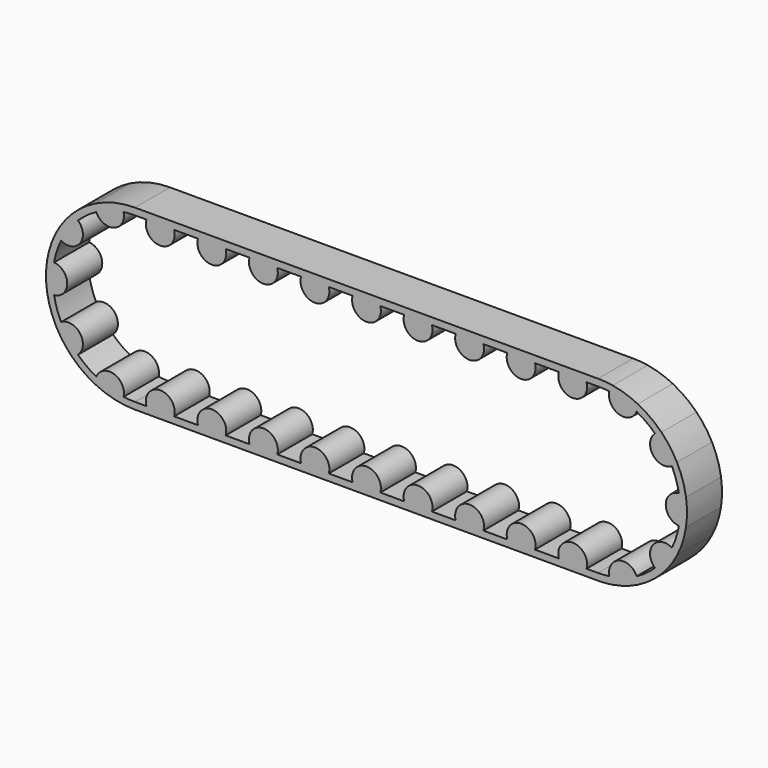
from build123d import *

# Parameters (mm, degrees)
F3_DEPTH = 25.4


with BuildPart() as f3:
    # F2 (on Front) → F3 (new body)
    with BuildSketch(Plane.XZ):
        with BuildLine():
            ThreePointArc((-6.5580901404, 47.171305671), (-3.2868824452, 47.5114410305), (0, 47.625))
            Line((0, 47.625), (6.6759446819, 47.625))
            ThreePointArc((6.6759446819, 47.625), (7.6523000339, 49.786472114), (9.1956373991, 51.5874))
            Line((9.1956373991, 51.5874), (0, 51.5874))
            ThreePointArc((0, 51.5874), (-4.2571154541, 51.4114462622), (-8.485190663, 50.8847853309))
            ThreePointArc((-8.485190663, 50.8847853309), (-7.2859359113, 49.1503637276), (-6.5580901404, 47.171305671))
        make_face()
        with BuildLine():
            ThreePointArc((9.1956373991, 51.5874), (7.6523000339, 49.786472114), (6.6759446819, 47.625))
            Line((6.6759446819, 47.625), (22.7579240323, 47.625))
            ThreePointArc((22.7579240323, 47.625), (21.7815686803, 49.786472114), (20.2382313151, 51.5874))
            Line((20.2382313151, 51.5874), (9.1956373991, 51.5874))
        make_face()
        with BuildLine():
            Line((22.7579240323, 47.625), (6.6759446819, 47.625))
            ThreePointArc((6.6759446819, 47.625), (14.7169343571, 36.9220438028), (22.7579240323, 47.625))
        make_face()
        with BuildLine():
            ThreePointArc((-22.4209914306, 42.0171366024), (-12.129837039, 37.3317997636), (-6.5580901404, 47.171305671))
            ThreePointArc((-6.5580901404, 47.171305671), (-14.7169343571, 45.2940665886), (-22.4209914306, 42.0171366024))
        make_face()
        with BuildLine():
            ThreePointArc((-22.4209914306, 42.0171366024), (-14.7169343571, 45.2940665886), (-6.5580901404, 47.171305671))
            ThreePointArc((-6.5580901404, 47.171305671), (-7.2859359113, 49.1503637276), (-8.485190663, 50.8847853309))
            ThreePointArc((-8.485190663, 50.8847853309), (-15.9413832956, 49.0625329287), (-23.0446629367, 46.1541260224))
            ThreePointArc((-23.0446629367, 46.1541260224), (-22.9954129717, 44.0460452131), (-22.4209914306, 42.0171366024))
        make_face()
        with BuildLine():
            ThreePointArc((20.2382313151, 51.5874), (21.7815686803, 49.786472114), (22.7579240323, 47.625))
            Line((22.7579240323, 47.625), (36.5771902535, 47.625))
            ThreePointArc((36.5771902535, 47.625), (37.5535456055, 49.786472114), (39.0968829707, 51.5874))
            Line((39.0968829707, 51.5874), (20.2382313151, 51.5874))
        make_face()
        with BuildLine():
            ThreePointArc((-33.032204179, 34.307639267), (-27.9932726404, 38.5294343571), (-22.4209914306, 42.0171366024))
            ThreePointArc((-22.4209914306, 42.0171366024), (-22.9954129717, 44.0460452131), (-23.0446629367, 46.1541260224))
            ThreePointArc((-23.0446629367, 46.1541260224), (-30.3223129241, 41.7350832956), (-36.7739898304, 36.1791861533))
            ThreePointArc((-36.7739898304, 36.1791861533), (-34.7843049161, 35.4809138575), (-33.032204179, 34.307639267))
        make_face()
        with BuildLine():
            ThreePointArc((39.0968829707, 51.5874), (37.5535456055, 49.786472114), (36.5771902535, 47.625))
            Line((36.5771902535, 47.625), (52.6591696039, 47.625))
            ThreePointArc((52.6591696039, 47.625), (51.6828142519, 49.786472114), (50.1394768867, 51.5874))
            Line((50.1394768867, 51.5874), (39.0968829707, 51.5874))
        make_face()
        with BuildLine():
            Line((52.6591696039, 47.625), (36.5771902535, 47.625))
            ThreePointArc((36.5771902535, 47.625), (44.6181799287, 36.9220438028), (52.6591696039, 47.625))
        make_face()
        with BuildLine():
            ThreePointArc((-42.8360163366, 20.8138494617), (-31.7563256461, 23.0723211151), (-33.032204179, 34.307639267))
            ThreePointArc((-33.032204179, 34.307639267), (-38.5294343571, 27.9932726404), (-42.8360163366, 20.8138494617))
        make_face()
        with BuildLine():
            ThreePointArc((-42.8360163366, 20.8138494617), (-38.5294343571, 27.9932726404), (-33.032204179, 34.307639267))
            ThreePointArc((-33.032204179, 34.307639267), (-34.7843049161, 35.4809138575), (-36.7739898304, 36.1791861533))
            ThreePointArc((-36.7739898304, 36.1791861533), (-41.7350832956, 30.3223129241), (-45.7722385539, 23.7941592944))
            ThreePointArc((-45.7722385539, 23.7941592944), (-44.4932956849, 22.1176344973), (-42.8360163366, 20.8138494617))
        make_face()
        with BuildLine():
            ThreePointArc((50.1394768867, 51.5874), (51.6828142519, 49.786472114), (52.6591696039, 47.625))
            Line((52.6591696039, 47.625), (66.478435825, 47.625))
            ThreePointArc((66.478435825, 47.625), (67.4547911771, 49.786472114), (68.9981285423, 51.5874))
            Line((68.9981285423, 51.5874), (50.1394768867, 51.5874))
        make_face()
        with BuildLine():
            ThreePointArc((-46.8891389446, 8.3396207368), (-45.2940665886, 14.7169343571), (-42.8360163366, 20.8138494617))
            ThreePointArc((-42.8360163366, 20.8138494617), (-44.4932956849, 22.1176344973), (-45.7722385539, 23.7941592944))
            ThreePointArc((-45.7722385539, 23.7941592944), (-49.0625329287, 15.9413832956), (-51.0163747846, 7.6543675504))
            ThreePointArc((-51.0163747846, 7.6543675504), (-48.9962517179, 8.2589608458), (-46.8891389446, 8.3396207368))
        make_face()
        with BuildLine():
            ThreePointArc((68.9981285423, 51.5874), (67.4547911771, 49.786472114), (66.478435825, 47.625))
            Line((66.478435825, 47.625), (82.5604151755, 47.625))
            ThreePointArc((82.5604151755, 47.625), (81.5840598235, 49.786472114), (80.0407224583, 51.5874))
            Line((80.0407224583, 51.5874), (68.9981285423, 51.5874))
        make_face()
        with BuildLine():
            Line((82.5604151755, 47.625), (66.478435825, 47.625))
            ThreePointArc((66.478435825, 47.625), (74.5194255003, 36.9220438028), (82.5604151755, 47.625))
        make_face()
        with BuildLine():
            ThreePointArc((-46.8891389446, -8.3396207368), (-39.2529772142, 0), (-46.8891389446, 8.3396207368))
            ThreePointArc((-46.8891389446, 8.3396207368), (-47.625, 0), (-46.8891389446, -8.3396207368))
        make_face()
        with BuildLine():
            ThreePointArc((-46.8891389446, -8.3396207368), (-47.625, 0), (-46.8891389446, 8.3396207368))
            ThreePointArc((-46.8891389446, 8.3396207368), (-48.9962517179, 8.2589608458), (-51.0163747846, 7.6543675504))
            ThreePointArc((-51.0163747846, 7.6543675504), (-51.5874, 0), (-51.0163747846, -7.6543675504))
            ThreePointArc((-51.0163747846, -7.6543675504), (-48.9962517179, -8.2589608458), (-46.8891389446, -8.3396207368))
        make_face()
        with BuildLine():
            ThreePointArc((80.0407224583, 51.5874), (81.5840598235, 49.786472114), (82.5604151755, 47.625))
            Line((82.5604151755, 47.625), (96.3796813966, 47.625))
            ThreePointArc((96.3796813966, 47.625), (97.3560367487, 49.786472114), (98.8993741139, 51.5874))
            Line((98.8993741139, 51.5874), (80.0407224583, 51.5874))
        make_face()
        with BuildLine():
            ThreePointArc((-42.8360163366, -20.8138494617), (-45.2940665886, -14.7169343571), (-46.8891389446, -8.3396207368))
            ThreePointArc((-46.8891389446, -8.3396207368), (-48.9962517179, -8.2589608458), (-51.0163747846, -7.6543675504))
            ThreePointArc((-51.0163747846, -7.6543675504), (-49.0625329287, -15.9413832956), (-45.7722385539, -23.7941592944))
            ThreePointArc((-45.7722385539, -23.7941592944), (-44.4932956849, -22.1176344973), (-42.8360163366, -20.8138494617))
        make_face()
        with BuildLine():
            ThreePointArc((98.8993741139, 51.5874), (97.3560367487, 49.786472114), (96.3796813966, 47.625))
            Line((96.3796813966, 47.625), (112.4616607471, 47.625))
            ThreePointArc((112.4616607471, 47.625), (111.485305395, 49.786472114), (109.9419680298, 51.5874))
            Line((109.9419680298, 51.5874), (98.8993741139, 51.5874))
        make_face()
        with BuildLine():
            Line((112.4616607471, 47.625), (96.3796813966, 47.625))
            ThreePointArc((96.3796813966, 47.625), (104.4206710719, 36.9220438028), (112.4616607471, 47.625))
        make_face()
        with BuildLine():
            ThreePointArc((-33.032204179, -34.307639267), (-31.7563256461, -23.0723211151), (-42.8360163366, -20.8138494617))
            ThreePointArc((-42.8360163366, -20.8138494617), (-38.5294343571, -27.9932726404), (-33.032204179, -34.307639267))
        make_face()
        with BuildLine():
            ThreePointArc((-33.032204179, -34.307639267), (-38.5294343571, -27.9932726404), (-42.8360163366, -20.8138494617))
            ThreePointArc((-42.8360163366, -20.8138494617), (-44.4932956849, -22.1176344973), (-45.7722385539, -23.7941592944))
            ThreePointArc((-45.7722385539, -23.7941592944), (-41.7350832956, -30.3223129241), (-36.7739898304, -36.1791861533))
            ThreePointArc((-36.7739898304, -36.1791861533), (-34.7843049161, -35.4809138575), (-33.032204179, -34.307639267))
        make_face()
        with BuildLine():
            ThreePointArc((109.9419680298, 51.5874), (111.485305395, 49.786472114), (112.4616607471, 47.625))
            Line((112.4616607471, 47.625), (126.2809269682, 47.625))
            ThreePointArc((126.2809269682, 47.625), (127.2572823202, 49.786472114), (128.8006196855, 51.5874))
            Line((128.8006196855, 51.5874), (109.9419680298, 51.5874))
        make_face()
        with BuildLine():
            ThreePointArc((-22.4209914306, -42.0171366024), (-27.9932726404, -38.5294343571), (-33.032204179, -34.307639267))
            ThreePointArc((-33.032204179, -34.307639267), (-34.7843049161, -35.4809138575), (-36.7739898304, -36.1791861533))
            ThreePointArc((-36.7739898304, -36.1791861533), (-30.3223129241, -41.7350832956), (-23.0446629367, -46.1541260224))
            ThreePointArc((-23.0446629367, -46.1541260224), (-22.9954129717, -44.0460452131), (-22.4209914306, -42.0171366024))
        make_face()
        with BuildLine():
            ThreePointArc((128.8006196855, 51.5874), (127.2572823202, 49.786472114), (126.2809269682, 47.625))
            Line((126.2809269682, 47.625), (142.3629063187, 47.625))
            ThreePointArc((142.3629063187, 47.625), (141.3865509666, 49.786472114), (139.8432136014, 51.5874))
            Line((139.8432136014, 51.5874), (128.8006196855, 51.5874))
        make_face()
        with BuildLine():
            Line((142.3629063187, 47.625), (126.2809269682, 47.625))
            ThreePointArc((126.2809269682, 47.625), (134.3219166434, 36.9220438028), (142.3629063187, 47.625))
        make_face()
        with BuildLine():
            ThreePointArc((-6.5580901404, -47.171305671), (-12.129837039, -37.3317997636), (-22.4209914306, -42.0171366024))
            ThreePointArc((-22.4209914306, -42.0171366024), (-14.7169343571, -45.2940665886), (-6.5580901404, -47.171305671))
        make_face()
        with BuildLine():
            ThreePointArc((-6.5580901404, -47.171305671), (-14.7169343571, -45.2940665886), (-22.4209914306, -42.0171366024))
            ThreePointArc((-22.4209914306, -42.0171366024), (-22.9954129717, -44.0460452131), (-23.0446629367, -46.1541260224))
            ThreePointArc((-23.0446629367, -46.1541260224), (-15.9413832956, -49.0625329287), (-8.485190663, -50.8847853309))
            ThreePointArc((-8.485190663, -50.8847853309), (-7.2859359113, -49.1503637276), (-6.5580901404, -47.171305671))
        make_face()
        with BuildLine():
            ThreePointArc((139.8432136014, 51.5874), (141.3865509666, 49.786472114), (142.3629063187, 47.625))
            Line((142.3629063187, 47.625), (156.1821725398, 47.625))
            ThreePointArc((156.1821725398, 47.625), (157.1585278918, 49.786472114), (158.701865257, 51.5874))
            Line((158.701865257, 51.5874), (139.8432136014, 51.5874))
        make_face()
        with BuildLine():
            ThreePointArc((0, -47.625), (-3.2868824452, -47.5114410305), (-6.5580901404, -47.171305671))
            ThreePointArc((-6.5580901404, -47.171305671), (-7.2859359113, -49.1503637276), (-8.485190663, -50.8847853309))
            ThreePointArc((-8.485190663, -50.8847853309), (-4.2571154541, -51.4114462622), (0, -51.5874))
            Line((0, -51.5874), (9.1956373991, -51.5874))
            ThreePointArc((9.1956373991, -51.5874), (7.6523000339, -49.786472114), (6.6759446819, -47.625))
            Line((6.6759446819, -47.625), (0, -47.625))
        make_face()
        with BuildLine():
            ThreePointArc((158.701865257, 51.5874), (157.1585278918, 49.786472114), (156.1821725398, 47.625))
            Line((156.1821725398, 47.625), (172.2641518903, 47.625))
            ThreePointArc((172.2641518903, 47.625), (171.2877965382, 49.786472114), (169.744459173, 51.5874))
            Line((169.744459173, 51.5874), (158.701865257, 51.5874))
        make_face()
        with BuildLine():
            Line((172.2641518903, 47.625), (156.1821725398, 47.625))
            ThreePointArc((156.1821725398, 47.625), (164.223162215, 36.9220438028), (172.2641518903, 47.625))
        make_face()
        with BuildLine():
            ThreePointArc((169.744459173, 51.5874), (171.2877965382, 49.786472114), (172.2641518903, 47.625))
            Line((172.2641518903, 47.625), (186.0834181114, 47.625))
            ThreePointArc((186.0834181114, 47.625), (187.0597734634, 49.786472114), (188.6031108286, 51.5874))
            Line((188.6031108286, 51.5874), (169.744459173, 51.5874))
        make_face()
        with BuildLine():
            ThreePointArc((22.7579240323, -47.625), (14.7169343571, -36.9220438028), (6.6759446819, -47.625))
            Line((6.6759446819, -47.625), (22.7579240323, -47.625))
        make_face()
        with BuildLine():
            Line((22.7579240323, -47.625), (6.6759446819, -47.625))
            ThreePointArc((6.6759446819, -47.625), (7.6523000339, -49.786472114), (9.1956373991, -51.5874))
            Line((9.1956373991, -51.5874), (20.2382313151, -51.5874))
            ThreePointArc((20.2382313151, -51.5874), (21.7815686803, -49.786472114), (22.7579240323, -47.625))
        make_face()
        with BuildLine():
            ThreePointArc((188.6031108286, 51.5874), (187.0597734634, 49.786472114), (186.0834181114, 47.625))
            Line((186.0834181114, 47.625), (202.1653974618, 47.625))
            Line((202.1653974618, 47.625), (215.984663683, 47.625))
            ThreePointArc((215.984663683, 47.625), (216.961019035, 49.786472114), (218.5043564002, 51.5874))
            Line((218.5043564002, 51.5874), (188.6031108286, 51.5874))
        make_face()
        with BuildLine():
            Line((202.1653974618, 47.625), (186.0834181114, 47.625))
            ThreePointArc((186.0834181114, 47.625), (194.1244077866, 36.9220438028), (202.1653974618, 47.625))
        make_face()
        with BuildLine():
            Line((36.5771902535, -47.625), (22.7579240323, -47.625))
            ThreePointArc((22.7579240323, -47.625), (21.7815686803, -49.786472114), (20.2382313151, -51.5874))
            Line((20.2382313151, -51.5874), (39.0968829707, -51.5874))
            ThreePointArc((39.0968829707, -51.5874), (37.5535456055, -49.786472114), (36.5771902535, -47.625))
        make_face()
        with BuildLine():
            ThreePointArc((52.6591696039, -47.625), (44.6181799287, -36.9220438028), (36.5771902535, -47.625))
            Line((36.5771902535, -47.625), (52.6591696039, -47.625))
        make_face()
        with BuildLine():
            Line((52.6591696039, -47.625), (36.5771902535, -47.625))
            ThreePointArc((36.5771902535, -47.625), (37.5535456055, -49.786472114), (39.0968829707, -51.5874))
            Line((39.0968829707, -51.5874), (50.1394768867, -51.5874))
            ThreePointArc((50.1394768867, -51.5874), (51.6828142519, -49.786472114), (52.6591696039, -47.625))
        make_face()
        with BuildLine():
            ThreePointArc((218.5043564002, 51.5874), (216.961019035, 49.786472114), (215.984663683, 47.625))
            Line((215.984663683, 47.625), (232.0666430334, 47.625))
            ThreePointArc((232.0666430334, 47.625), (231.0902876814, 49.786472114), (229.5469503162, 51.5874))
            Line((229.5469503162, 51.5874), (218.5043564002, 51.5874))
        make_face()
        with BuildLine():
            Line((232.0666430334, 47.625), (215.984663683, 47.625))
            ThreePointArc((215.984663683, 47.625), (224.0256533582, 36.9220438028), (232.0666430334, 47.625))
        make_face()
        with BuildLine():
            Line((66.478435825, -47.625), (52.6591696039, -47.625))
            ThreePointArc((52.6591696039, -47.625), (51.6828142519, -49.786472114), (50.1394768867, -51.5874))
            Line((50.1394768867, -51.5874), (68.9981285423, -51.5874))
            ThreePointArc((68.9981285423, -51.5874), (67.4547911771, -49.786472114), (66.478435825, -47.625))
        make_face()
        with BuildLine():
            ThreePointArc((229.5469503162, 51.5874), (231.0902876814, 49.786472114), (232.0666430334, 47.625))
            Line((232.0666430334, 47.625), (245.8859092545, 47.625))
            ThreePointArc((245.8859092545, 47.625), (246.8622646066, 49.786472114), (248.4056019718, 51.5874))
            Line((248.4056019718, 51.5874), (229.5469503162, 51.5874))
        make_face()
        with BuildLine():
            ThreePointArc((82.5604151755, -47.625), (74.5194255003, -36.9220438028), (66.478435825, -47.625))
            Line((66.478435825, -47.625), (82.5604151755, -47.625))
        make_face()
        with BuildLine():
            Line((82.5604151755, -47.625), (66.478435825, -47.625))
            ThreePointArc((66.478435825, -47.625), (67.4547911771, -49.786472114), (68.9981285423, -51.5874))
            Line((68.9981285423, -51.5874), (80.0407224583, -51.5874))
            ThreePointArc((80.0407224583, -51.5874), (81.5840598235, -49.786472114), (82.5604151755, -47.625))
        make_face()
        with BuildLine():
            ThreePointArc((248.4056019718, 51.5874), (246.8622646066, 49.786472114), (245.8859092545, 47.625))
            Line((245.8859092545, 47.625), (261.967888605, 47.625))
            ThreePointArc((261.967888605, 47.625), (260.991533253, 49.786472114), (259.4481958878, 51.5874))
            Line((259.4481958878, 51.5874), (248.4056019718, 51.5874))
        make_face()
        with BuildLine():
            Line((261.967888605, 47.625), (245.8859092545, 47.625))
            ThreePointArc((245.8859092545, 47.625), (253.9268989298, 36.9220438028), (261.967888605, 47.625))
        make_face()
        with BuildLine():
            Line((96.3796813966, -47.625), (82.5604151755, -47.625))
            ThreePointArc((82.5604151755, -47.625), (81.5840598235, -49.786472114), (80.0407224583, -51.5874))
            Line((80.0407224583, -51.5874), (98.8993741139, -51.5874))
            ThreePointArc((98.8993741139, -51.5874), (97.3560367487, -49.786472114), (96.3796813966, -47.625))
        make_face()
        with BuildLine():
            ThreePointArc((259.4481958878, 51.5874), (260.991533253, 49.786472114), (261.967888605, 47.625))
            Line((261.967888605, 47.625), (268.6438332869, 47.625))
            ThreePointArc((268.6438332869, 47.625), (271.930715732, 47.5114410305), (275.2019234272, 47.171305671))
            ThreePointArc((275.2019234272, 47.171305671), (275.9297691982, 49.1503637276), (277.1290239498, 50.8847853309))
            ThreePointArc((277.1290239498, 50.8847853309), (272.900948741, 51.4114462622), (268.6438332869, 51.5874))
            Line((268.6438332869, 51.5874), (259.4481958878, 51.5874))
        make_face()
        with BuildLine():
            ThreePointArc((112.4616607471, -47.625), (104.4206710719, -36.9220438028), (96.3796813966, -47.625))
            Line((96.3796813966, -47.625), (112.4616607471, -47.625))
        make_face()
        with BuildLine():
            Line((112.4616607471, -47.625), (96.3796813966, -47.625))
            ThreePointArc((96.3796813966, -47.625), (97.3560367487, -49.786472114), (98.8993741139, -51.5874))
            Line((98.8993741139, -51.5874), (109.9419680298, -51.5874))
            ThreePointArc((109.9419680298, -51.5874), (111.485305395, -49.786472114), (112.4616607471, -47.625))
        make_face()
        with BuildLine():
            Line((126.2809269682, -47.625), (112.4616607471, -47.625))
            ThreePointArc((112.4616607471, -47.625), (111.485305395, -49.786472114), (109.9419680298, -51.5874))
            Line((109.9419680298, -51.5874), (128.8006196855, -51.5874))
            ThreePointArc((128.8006196855, -51.5874), (127.2572823202, -49.786472114), (126.2809269682, -47.625))
        make_face()
        with BuildLine():
            ThreePointArc((277.1290239498, 50.8847853309), (275.9297691982, 49.1503637276), (275.2019234272, 47.171305671))
            ThreePointArc((275.2019234272, 47.171305671), (283.360767644, 45.2940665886), (291.0648247175, 42.0171366024))
            ThreePointArc((291.0648247175, 42.0171366024), (291.6392462586, 44.0460452131), (291.6884962236, 46.1541260224))
            ThreePointArc((291.6884962236, 46.1541260224), (284.5852165825, 49.0625329287), (277.1290239498, 50.8847853309))
        make_face()
        with BuildLine():
            ThreePointArc((291.0648247175, 42.0171366024), (283.360767644, 45.2940665886), (275.2019234272, 47.171305671))
            ThreePointArc((275.2019234272, 47.171305671), (280.7736703259, 37.3317997636), (291.0648247175, 42.0171366024))
        make_face()
        with BuildLine():
            ThreePointArc((142.3629063187, -47.625), (134.3219166434, -36.9220438028), (126.2809269682, -47.625))
            Line((126.2809269682, -47.625), (142.3629063187, -47.625))
        make_face()
        with BuildLine():
            Line((142.3629063187, -47.625), (126.2809269682, -47.625))
            ThreePointArc((126.2809269682, -47.625), (127.2572823202, -49.786472114), (128.8006196855, -51.5874))
            Line((128.8006196855, -51.5874), (139.8432136014, -51.5874))
            ThreePointArc((139.8432136014, -51.5874), (141.3865509666, -49.786472114), (142.3629063187, -47.625))
        make_face()
        with BuildLine():
            ThreePointArc((291.6884962236, 46.1541260224), (291.6392462586, 44.0460452131), (291.0648247175, 42.0171366024))
            ThreePointArc((291.0648247175, 42.0171366024), (296.6371059273, 38.5294343571), (301.6760374659, 34.307639267))
            ThreePointArc((301.6760374659, 34.307639267), (303.4281382029, 35.4809138575), (305.4178231173, 36.1791861533))
            ThreePointArc((305.4178231173, 36.1791861533), (298.966146211, 41.7350832956), (291.6884962236, 46.1541260224))
        make_face()
        with BuildLine():
            Line((156.1821725398, -47.625), (142.3629063187, -47.625))
            ThreePointArc((142.3629063187, -47.625), (141.3865509666, -49.786472114), (139.8432136014, -51.5874))
            Line((139.8432136014, -51.5874), (158.701865257, -51.5874))
            ThreePointArc((158.701865257, -51.5874), (157.1585278918, -49.786472114), (156.1821725398, -47.625))
        make_face()
        with BuildLine():
            ThreePointArc((305.4178231173, 36.1791861533), (303.4281382029, 35.4809138575), (301.6760374659, 34.307639267))
            ThreePointArc((301.6760374659, 34.307639267), (307.173267644, 27.9932726404), (311.4798496235, 20.8138494617))
            ThreePointArc((311.4798496235, 20.8138494617), (313.1371289717, 22.1176344973), (314.4160718408, 23.7941592944))
            ThreePointArc((314.4160718408, 23.7941592944), (310.3789165825, 30.3223129241), (305.4178231173, 36.1791861533))
        make_face()
        with BuildLine():
            ThreePointArc((311.4798496235, 20.8138494617), (307.173267644, 27.9932726404), (301.6760374659, 34.307639267))
            ThreePointArc((301.6760374659, 34.307639267), (300.400158933, 23.0723211151), (311.4798496235, 20.8138494617))
        make_face()
        with BuildLine():
            ThreePointArc((172.2641518903, -47.625), (164.223162215, -36.9220438028), (156.1821725398, -47.625))
            Line((156.1821725398, -47.625), (172.2641518903, -47.625))
        make_face()
        with BuildLine():
            Line((172.2641518903, -47.625), (156.1821725398, -47.625))
            ThreePointArc((156.1821725398, -47.625), (157.1585278918, -49.786472114), (158.701865257, -51.5874))
            Line((158.701865257, -51.5874), (169.744459173, -51.5874))
            ThreePointArc((169.744459173, -51.5874), (171.2877965382, -49.786472114), (172.2641518903, -47.625))
        make_face()
        with BuildLine():
            ThreePointArc((314.4160718408, 23.7941592944), (313.1371289717, 22.1176344973), (311.4798496235, 20.8138494617))
            ThreePointArc((311.4798496235, 20.8138494617), (313.9378998754, 14.7169343571), (315.5329722315, 8.3396207368))
            ThreePointArc((315.5329722315, 8.3396207368), (317.6400850048, 8.2589608458), (319.6602080715, 7.6543675504))
            ThreePointArc((319.6602080715, 7.6543675504), (317.7063662156, 15.9413832956), (314.4160718408, 23.7941592944))
        make_face()
        with BuildLine():
            Line((186.0834181114, -47.625), (172.2641518903, -47.625))
            ThreePointArc((172.2641518903, -47.625), (171.2877965382, -49.786472114), (169.744459173, -51.5874))
            Line((169.744459173, -51.5874), (188.6031108286, -51.5874))
            ThreePointArc((188.6031108286, -51.5874), (187.0597734634, -49.786472114), (186.0834181114, -47.625))
        make_face()
        with BuildLine():
            ThreePointArc((319.6602080715, 7.6543675504), (317.6400850048, 8.2589608458), (315.5329722315, 8.3396207368))
            ThreePointArc((315.5329722315, 8.3396207368), (316.2688332869, 0), (315.5329722315, -8.3396207368))
            ThreePointArc((315.5329722315, -8.3396207368), (317.6400850048, -8.2589608458), (319.6602080715, -7.6543675504))
            ThreePointArc((319.6602080715, -7.6543675504), (320.2312332869, 0), (319.6602080715, 7.6543675504))
        make_face()
        with BuildLine():
            ThreePointArc((315.5329722315, -8.3396207368), (316.2688332869, 0), (315.5329722315, 8.3396207368))
            ThreePointArc((315.5329722315, 8.3396207368), (307.8968105011, 0), (315.5329722315, -8.3396207368))
        make_face()
        with BuildLine():
            ThreePointArc((202.1653974618, -47.625), (194.1244077866, -36.9220438028), (186.0834181114, -47.625))
            Line((186.0834181114, -47.625), (202.1653974618, -47.625))
        make_face()
        with BuildLine():
            Line((202.1653974618, -47.625), (186.0834181114, -47.625))
            ThreePointArc((186.0834181114, -47.625), (187.0597734634, -49.786472114), (188.6031108286, -51.5874))
            Line((188.6031108286, -51.5874), (199.6457047446, -51.5874))
            ThreePointArc((199.6457047446, -51.5874), (201.1890421098, -49.786472114), (202.1653974618, -47.625))
        make_face()
        with BuildLine():
            ThreePointArc((319.6602080715, -7.6543675504), (317.6400850048, -8.2589608458), (315.5329722315, -8.3396207368))
            ThreePointArc((315.5329722315, -8.3396207368), (313.9378998754, -14.7169343571), (311.4798496235, -20.8138494617))
            ThreePointArc((311.4798496235, -20.8138494617), (313.1371289717, -22.1176344973), (314.4160718408, -23.7941592944))
            ThreePointArc((314.4160718408, -23.7941592944), (317.7063662156, -15.9413832956), (319.6602080715, -7.6543675504))
        make_face()
        with BuildLine():
            Line((215.984663683, -47.625), (202.1653974618, -47.625))
            ThreePointArc((202.1653974618, -47.625), (201.1890421098, -49.786472114), (199.6457047446, -51.5874))
            Line((199.6457047446, -51.5874), (218.5043564002, -51.5874))
            ThreePointArc((218.5043564002, -51.5874), (216.961019035, -49.786472114), (215.984663683, -47.625))
        make_face()
        with BuildLine():
            ThreePointArc((314.4160718408, -23.7941592944), (313.1371289717, -22.1176344973), (311.4798496235, -20.8138494617))
            ThreePointArc((311.4798496235, -20.8138494617), (307.173267644, -27.9932726404), (301.6760374659, -34.307639267))
            ThreePointArc((301.6760374659, -34.307639267), (303.4281382029, -35.4809138575), (305.4178231173, -36.1791861533))
            ThreePointArc((305.4178231173, -36.1791861533), (310.3789165825, -30.3223129241), (314.4160718408, -23.7941592944))
        make_face()
        with BuildLine():
            ThreePointArc((301.6760374659, -34.307639267), (307.173267644, -27.9932726404), (311.4798496235, -20.8138494617))
            ThreePointArc((311.4798496235, -20.8138494617), (300.400158933, -23.0723211151), (301.6760374659, -34.307639267))
        make_face()
        with BuildLine():
            ThreePointArc((232.0666430334, -47.625), (224.0256533582, -36.9220438028), (215.984663683, -47.625))
            Line((215.984663683, -47.625), (232.0666430334, -47.625))
        make_face()
        with BuildLine():
            Line((232.0666430334, -47.625), (215.984663683, -47.625))
            ThreePointArc((215.984663683, -47.625), (216.961019035, -49.786472114), (218.5043564002, -51.5874))
            Line((218.5043564002, -51.5874), (229.5469503162, -51.5874))
            ThreePointArc((229.5469503162, -51.5874), (231.0902876814, -49.786472114), (232.0666430334, -47.625))
        make_face()
        with BuildLine():
            ThreePointArc((305.4178231173, -36.1791861533), (303.4281382029, -35.4809138575), (301.6760374659, -34.307639267))
            ThreePointArc((301.6760374659, -34.307639267), (296.6371059273, -38.5294343571), (291.0648247175, -42.0171366024))
            ThreePointArc((291.0648247175, -42.0171366024), (291.6392462586, -44.0460452131), (291.6884962236, -46.1541260224))
            ThreePointArc((291.6884962236, -46.1541260224), (298.966146211, -41.7350832956), (305.4178231173, -36.1791861533))
        make_face()
        with BuildLine():
            Line((245.8859092545, -47.625), (232.0666430334, -47.625))
            ThreePointArc((232.0666430334, -47.625), (231.0902876814, -49.786472114), (229.5469503162, -51.5874))
            Line((229.5469503162, -51.5874), (248.4056019718, -51.5874))
            ThreePointArc((248.4056019718, -51.5874), (246.8622646066, -49.786472114), (245.8859092545, -47.625))
        make_face()
        with BuildLine():
            ThreePointArc((291.6884962236, -46.1541260224), (291.6392462586, -44.0460452131), (291.0648247175, -42.0171366024))
            ThreePointArc((291.0648247175, -42.0171366024), (283.360767644, -45.2940665886), (275.2019234272, -47.171305671))
            ThreePointArc((275.2019234272, -47.171305671), (275.9297691982, -49.1503637276), (277.1290239498, -50.8847853309))
            ThreePointArc((277.1290239498, -50.8847853309), (284.5852165825, -49.0625329287), (291.6884962236, -46.1541260224))
        make_face()
        with BuildLine():
            ThreePointArc((275.2019234272, -47.171305671), (283.360767644, -45.2940665886), (291.0648247175, -42.0171366024))
            ThreePointArc((291.0648247175, -42.0171366024), (280.7736703259, -37.3317997636), (275.2019234272, -47.171305671))
        make_face()
        with BuildLine():
            ThreePointArc((261.967888605, -47.625), (253.9268989298, -36.9220438028), (245.8859092545, -47.625))
            Line((245.8859092545, -47.625), (261.967888605, -47.625))
        make_face()
        with BuildLine():
            Line((261.967888605, -47.625), (245.8859092545, -47.625))
            ThreePointArc((245.8859092545, -47.625), (246.8622646066, -49.786472114), (248.4056019718, -51.5874))
            Line((248.4056019718, -51.5874), (259.4481958878, -51.5874))
            ThreePointArc((259.4481958878, -51.5874), (260.991533253, -49.786472114), (261.967888605, -47.625))
        make_face()
        with BuildLine():
            ThreePointArc((277.1290239498, -50.8847853309), (275.9297691982, -49.1503637276), (275.2019234272, -47.171305671))
            ThreePointArc((275.2019234272, -47.171305671), (271.930715732, -47.5114410305), (268.6438332869, -47.625))
            Line((268.6438332869, -47.625), (261.967888605, -47.625))
            ThreePointArc((261.967888605, -47.625), (260.991533253, -49.786472114), (259.4481958878, -51.5874))
            Line((259.4481958878, -51.5874), (268.6438332869, -51.5874))
            ThreePointArc((268.6438332869, -51.5874), (272.900948741, -51.4114462622), (277.1290239498, -50.8847853309))
        make_face()
    extrude(amount=F3_DEPTH)


solid = f3.part
